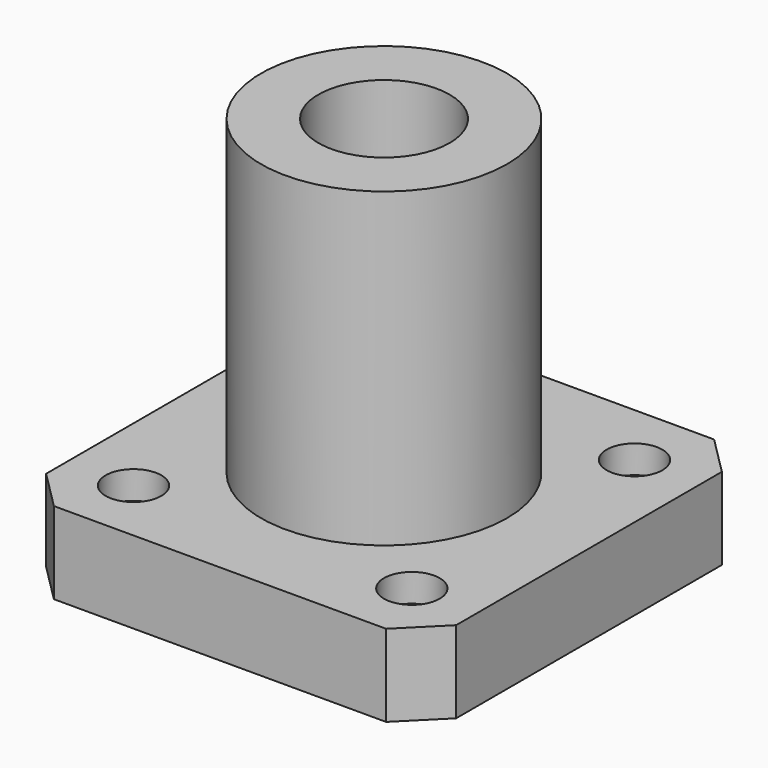
from build123d import *

# Parameters (mm, degrees)
F0_W     = 25
F0_H     = 25
F0_R     = 1.7
F0_R_2   = 7.5
F0_R_3   = 4
F1_DEPTH = 3.3
F2_DEPTH = 1.7
F3_R     = 7.5
F3_R_2   = 4
F4_DEPTH = 19
F6_DEPTH = 25
F7_R     = 3.25
F7_R_2   = 1.7
F8_DEPTH = 3.3


# Not quite as in the source:
# - a feature names something its author has since deleted; it is built from what else it names


with BuildPart() as f1:
    # F0 (on Top) → F1 (new body)
    with BuildSketch(Plane.XY):
        Rectangle(F0_W, F0_H)
        with Locations((-8.4852813742, -8.4852813742)):
            Circle(F0_R, mode=Mode.SUBTRACT)
        with Locations((8.4852813742, -8.4852813742)):
            Circle(F0_R, mode=Mode.SUBTRACT)
        with Locations((-8.4852813742, 8.4852813742)):
            Circle(F0_R, mode=Mode.SUBTRACT)
        Circle(F0_R_2, mode=Mode.SUBTRACT)
        with Locations((8.4852813742, 8.4852813742)):
            Circle(F0_R, mode=Mode.SUBTRACT)
        Circle(F0_R_2)
        Circle(F0_R_3, mode=Mode.SUBTRACT)
    extrude(amount=-F1_DEPTH)

    # F0 (on Top) → F2 (join)
    with BuildSketch(Plane.XY):
        Rectangle(F0_W, F0_H)
        with Locations((-8.4852813742, -8.4852813742)):
            Circle(F0_R, mode=Mode.SUBTRACT)
        with Locations((8.4852813742, -8.4852813742)):
            Circle(F0_R, mode=Mode.SUBTRACT)
        with Locations((-8.4852813742, 8.4852813742)):
            Circle(F0_R, mode=Mode.SUBTRACT)
        Circle(F0_R_2, mode=Mode.SUBTRACT)
        with Locations((8.4852813742, 8.4852813742)):
            Circle(F0_R, mode=Mode.SUBTRACT)
        Circle(F0_R_2)
        Circle(F0_R_3, mode=Mode.SUBTRACT)
    extrude(amount=F2_DEPTH)

    # F3 (on face) → F4 (join)
    with BuildSketch(Plane.XY.offset(1.7)):
        Circle(F3_R)
        Circle(F3_R_2, mode=Mode.SUBTRACT)
    extrude(amount=F4_DEPTH)

    # F5 (on face) → F6 (cut)
    with BuildSketch(Plane.XY.offset(1.7)):
        Polygon((-12.5, 12.5), (-12.5, 10.127416998), (-10.127416998, 12.5), align=None)
        Polygon((-10.127416998, -12.5), (-12.5, -10.127416998), (-12.5, -12.5), align=None)
        Polygon((12.5, -10.127416998), (10.127416998, -12.5), (12.5, -12.5), align=None)
        Polygon((12.5, 12.5), (10.127416998, 12.5), (12.5, 10.127416998), align=None)
    extrude(amount=-F6_DEPTH, mode=Mode.SUBTRACT)

    # F7 (on face) → F8 (cut)
    with BuildSketch(Plane(origin=(0, 0, -3.3), x_dir=(1, 0, 0), z_dir=(0, 0, -1))):
        with Locations((-8.4852813742, 8.4852813742)):
            Circle(F7_R)
        with Locations((-8.4852813742, 8.4852813742)):
            Circle(F7_R_2, mode=Mode.SUBTRACT)
        with Locations((8.4852813742, 8.4852813742)):
            Circle(F7_R)
        with Locations((8.4852813742, 8.4852813742)):
            Circle(F7_R_2, mode=Mode.SUBTRACT)
        with Locations((-8.4852813742, -8.4852813742)):
            Circle(F7_R)
        with Locations((-8.4852813742, -8.4852813742)):
            Circle(F7_R_2, mode=Mode.SUBTRACT)
        with Locations((8.4852813742, -8.4852813742)):
            Circle(F7_R)
        with Locations((8.4852813742, -8.4852813742)):
            Circle(F7_R_2, mode=Mode.SUBTRACT)
    extrude(amount=-F8_DEPTH, mode=Mode.SUBTRACT)


solid = f1.part
